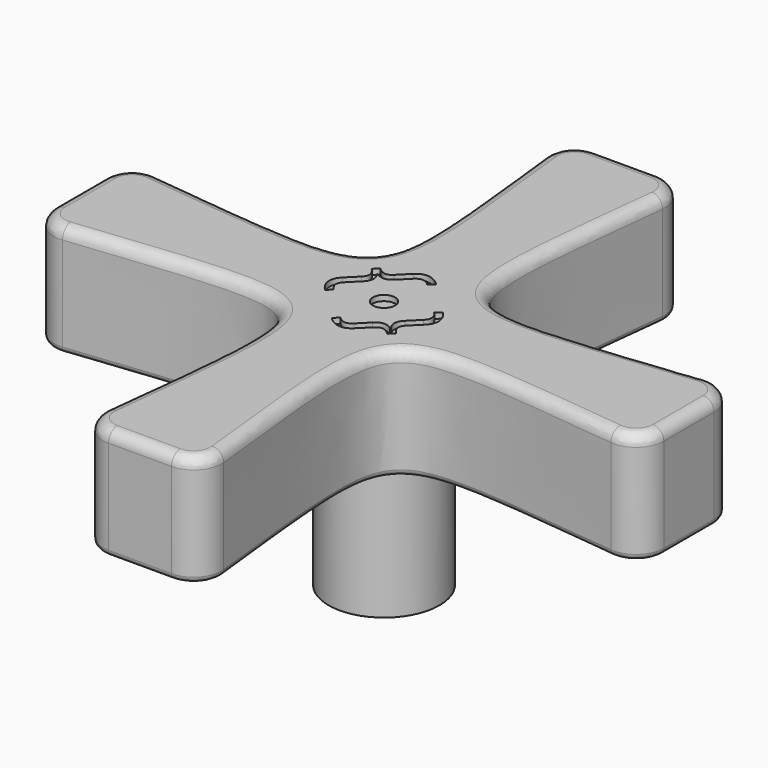
from build123d import *

# Parameters (mm, degrees)
F1_DEPTH     = 12.7
F2_R         = 6.35
F3_DEPTH     = 15.875
F4_R         = 1.27
F4_TEXT_SIZE = 11.4652777778
F5_DEPTH     = 0.635
F6_R         = 3.175
F7_R         = 1.27
F8_R         = 0.635


# Not quite as in the source:
# - Text() gives the source's letters only with a copy of the font that has no kerning and outlines rounded to 1/6400 em; it was checked with that copy


with BuildPart() as f1:
    # F0 (on Top) → F1 (new body)
    with BuildSketch(Plane.XY):
        with BuildLine():
            add(Edge.make_bspline(
                [(-34.925, 7.14375), (-15.875, 5.08), (-2.9928841816, 2.9928841816), (-5.08, 15.875), (-7.14375, 34.925)],
                knots=[0, 0, 0, 0, 0.5, 1, 1, 1, 1], degree=3))
            Line((-34.925, 7.14375), (-34.925, -7.14375))
            add(Edge.make_bspline(
                [(-34.925, -7.14375), (-15.875, -5.08), (-2.9928841816, -2.9928841816), (-5.08, -15.875), (-7.14375, -34.925)],
                knots=[0, 0, 0, 0, 0.5, 1, 1, 1, 1], degree=3))
            Line((-7.14375, -34.925), (7.14375, -34.925))
            add(Edge.make_bspline(
                [(34.925, -7.14375), (15.875, -5.08), (2.9928841816, -2.9928841816), (5.08, -15.875), (7.14375, -34.925)],
                knots=[0, 0, 0, 0, 0.5, 1, 1, 1, 1], degree=3))
            Line((34.925, -7.14375), (34.925, 7.14375))
            add(Edge.make_bspline(
                [(34.925, 7.14375), (15.875, 5.08), (2.9928841816, 2.9928841816), (5.08, 15.875), (7.14375, 34.925)],
                knots=[0, 0, 0, 0, 0.5, 1, 1, 1, 1], degree=3))
            Line((7.14375, 34.925), (-7.14375, 34.925))
        make_face()
    extrude(amount=F1_DEPTH)

    # F2 (on face) → F3 (join)
    with BuildSketch(Plane(origin=(0, 0, 0), x_dir=(1, 0, 0), z_dir=(0, 0, -1))):
        Circle(F2_R)
    extrude(amount=F3_DEPTH)

    # F4 (on face) → F5 (cut)
    with BuildSketch(Plane.XY.offset(12.7)):
        Circle(F4_R)
        with Locations(Location((-7.0171695658, 2.5089796451), (0, 0, -45))):
            Text('{', F4_TEXT_SIZE, font='Open Sans', text_align=(TextAlign.LEFT, TextAlign.BOTTOM))
        with Locations(Location((-0.6528280204, -3.8553619003), (0, 0, -45))):
            Text('}', F4_TEXT_SIZE, font='Open Sans', text_align=(TextAlign.LEFT, TextAlign.BOTTOM))
    extrude(amount=-F5_DEPTH, mode=Mode.SUBTRACT)

    # F6
    f6_edges = [f1.edges().sort_by_distance(p)[0] for p in [
        (7.14375, -34.925, 6.35),
        (34.925, -7.14375, 6.35),
        (34.925, 7.14375, 6.35),
        (7.14375, 34.925, 6.35),
        (-7.14375, 34.925, 6.35),
        (-34.925, -7.14375, 6.35),
        (-34.925, 7.14375, 6.35),
        (-7.14375, -34.925, 6.35),
    ]]
    fillet(f6_edges, radius=F6_R)

    # F7
    f7_edges = [f1.edges().sort_by_distance(p)[0] for p in [
        (-6.735192, -6.735192, 12.7),
        (-6.735192, 6.735192, 12.7),
        (-33.868764, 5.967534, 12.7),
        (-5.967534, 33.868764, 12.7),
        (-34.925, 0, 12.7),
        (0, 34.925, 12.7),
        (-33.868764, -5.967534, 12.7),
        (5.967534, 33.868764, 12.7),
        (6.735192, 6.735192, 12.7),
        (-5.967534, -33.868764, 12.7),
        (33.868764, 5.967534, 12.7),
        (0, -34.925, 12.7),
        (34.925, 0, 12.7),
        (5.967534, -33.868764, 12.7),
        (33.868764, -5.967534, 12.7),
        (6.735192, -6.735192, 12.7),
    ]]
    fillet(f7_edges, radius=F7_R)

    # F8
    f8_edges = [f1.edges().sort_by_distance(p)[0] for p in [
        (-6.735192, 6.735192, 0),
        (-33.868764, 5.967534, 0),
        (-5.967534, 33.868764, 0),
        (-34.925, 0, 0),
        (0, 34.925, 0),
        (-33.868764, -5.967534, 0),
        (5.967534, 33.868764, 0),
        (-6.735192, -6.735192, 0),
        (6.735192, 6.735192, 0),
        (-5.967534, -33.868764, 0),
        (33.868764, 5.967534, 0),
        (0, -34.925, 0),
        (34.925, 0, 0),
        (5.967534, -33.868764, 0),
        (33.868764, -5.967534, 0),
        (6.735192, -6.735192, 0),
    ]]
    fillet(f8_edges, radius=F8_R)


solid = f1.part
